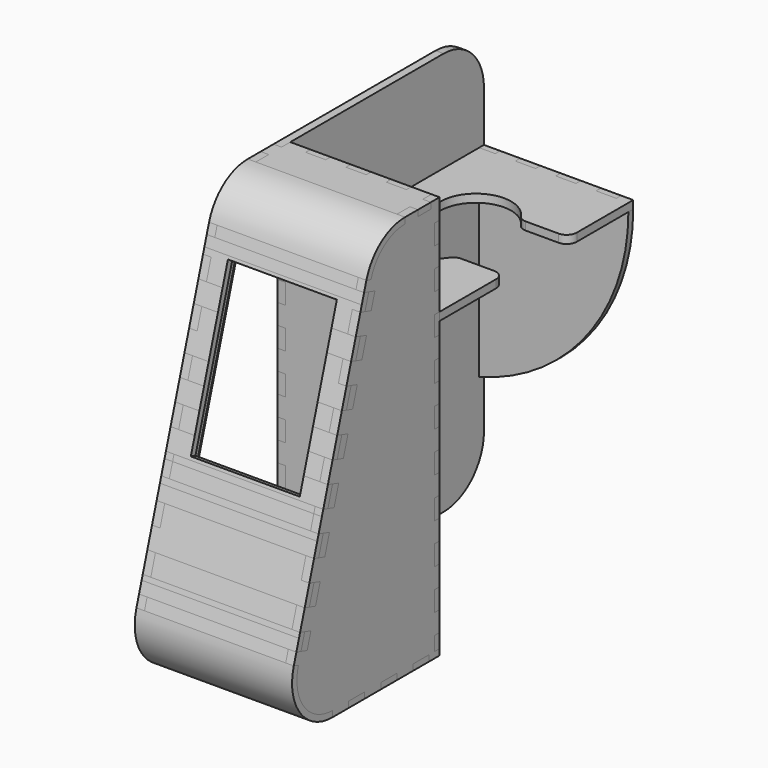
from build123d import *

# Parameters (mm, degrees)
F0_W      = 3
F0_H      = 7
F0_H_2    = 10
F0_R      = 2
F0_W_2    = 10
F0_H_3    = 4
F0_H_4    = 3
F0_W_3    = 2.3992337277
F0_W_4    = 3.3992337277
F1_DEPTH  = 4
F2_DEPTH  = 78
F3_DEPTH  = 78
F0_W_5    = 8
F4_DEPTH  = 78
F5_DEPTH  = 78
F6_START  = 74
F6_DEPTH  = 4
F7_W      = 57
F7_H      = 86.0071991074
F7_W_2    = 54
F7_H_2    = 80.0071991074
F7_W_3    = 59.9
F7_H_3    = 39.3927373791
F8_DEPTH  = 4
F9_DEPTH  = 3
F15_W     = 10
F15_H     = 3
F15_H_2   = 4
F16_DEPTH = 3
F19_W     = 4
F19_H     = 15
F19_H_2   = 10
F19_H_3   = 11
F20_DEPTH = 3
F21_DEPTH = 4
F24_R     = 4
F25_DEPTH = 3
F27_DEPTH = 4


# Not quite as in the source:
# - a feature names something its author has since deleted; it is built from what else it names


with BuildPart() as f1:
    # F0 (on Right) → F1 (new body)
    with BuildSketch(Plane.YZ):
        Polygon((-63.4476184856, 111.4009652057), (-66.3210973413, 112.2630088624), (-69.194576197, 102.6847460101), (-66.3210973413, 101.8227023534), align=None)
        Polygon((-66.3210973413, 101.8227023534), (-62.4897922004, 100.6733108112), (-59.6163133447, 110.2515736634), (-63.4476184856, 111.4009652057), align=None)
        Polygon((-53.8693556334, 129.4080993678), (-57.7006607743, 130.5574909101), (-60.57413963, 120.9792280579), (-56.7428344891, 119.8298365156), align=None)
        Polygon((-51.953703063, 149.7140166145), (-54.8271819186, 150.5760602712), (-57.7006607743, 140.997797419), (-54.8271819186, 140.1357537623), align=None)
        Polygon((-48.1223979221, 148.5646250722), (-51.953703063, 149.7140166145), (-54.8271819186, 140.1357537623), (-50.9958767778, 138.98636222), align=None)
        Polygon((-46.2067453516, 168.8705423189), (-49.0802242073, 169.7325859756), (-51.953703063, 160.1543231234), (-49.0802242073, 159.2922794667), align=None)
        Polygon((-42.3754402108, 167.7211507767), (-46.2067453516, 168.8705423189), (-49.0802242073, 159.2922794667), (-45.2489190664, 158.1428879244), align=None)
        Polygon((-13.3992337277, 197), (-13.3992337277, 200), (-21.3992337277, 200), (-21.3992337277, 198.5), (-21.3992337277, 197), align=None)
        with Locations((-1.5, 193.5)):
            Rectangle(F0_W, F0_H)
        with Locations((-1.5, 175)):
            Rectangle(F0_W, F0_H_2)
        with Locations((-1.5, 155)):
            Rectangle(F0_W, F0_H_2)
        with Locations((-1.5, 135)):
            Rectangle(F0_W, F0_H_2)
        with Locations((-1.5, 115)):
            Rectangle(F0_W, F0_H_2)
        with Locations((-1.5, 95)):
            Rectangle(F0_W, F0_H_2)
        with Locations((-1.5, 75)):
            Rectangle(F0_W, F0_H_2)
        with Locations((-1.5, 55)):
            Rectangle(F0_W, F0_H_2)
        with Locations((-1.5, 35)):
            Rectangle(F0_W, F0_H_2)
        with Locations((-1.5, 15)):
            Rectangle(F0_W, F0_H_2)
        with BuildLine():
            Line((0, 3), (0, 0))
            Line((0, 0), (95, 0))
            ThreePointArc((95, 0), (112.6776695297, 7.3223304703), (120, 25))
            Line((120, 25), (120, 175))
            ThreePointArc((120, 175), (112.6776695297, 192.6776695297), (95, 200))
            Line((95, 200), (0, 200))
            Line((0, 200), (0, 197))
            Line((0, 197), (0, 190))
            Line((0, 190), (0, 180))
            Line((0, 180), (0, 170))
            Line((0, 170), (0, 160))
            Line((0, 160), (0, 150))
            Line((0, 150), (0, 140))
            Line((0, 140), (0, 130))
            Line((0, 130), (0, 120))
            Line((0, 120), (0, 110))
            Line((0, 110), (0, 100))
            Line((0, 100), (0, 90))
            Line((0, 90), (0, 80))
            Line((0, 80), (0, 70))
            Line((0, 70), (0, 60))
            Line((0, 60), (0, 50))
            Line((0, 50), (0, 40))
            Line((0, 40), (0, 30))
            Line((0, 30), (0, 20))
            Line((0, 20), (0, 10))
            Line((0, 10), (0, 3))
        make_face()
        with Locations((95, 25)):
            Circle(F0_R, mode=Mode.SUBTRACT)
        with Locations((10, 148)):
            Rectangle(F0_W_2, F0_H_3, mode=Mode.SUBTRACT)
        with Locations((30, 148)):
            Rectangle(F0_W_2, F0_H_3, mode=Mode.SUBTRACT)
        with Locations((50, 148)):
            Rectangle(F0_W_2, F0_H_3, mode=Mode.SUBTRACT)
        with Locations((70, 148)):
            Rectangle(F0_W_2, F0_H_3, mode=Mode.SUBTRACT)
        with Locations((90, 148)):
            Rectangle(F0_W_2, F0_H_3, mode=Mode.SUBTRACT)
        with Locations((110, 148)):
            Rectangle(F0_W_2, F0_H_3, mode=Mode.SUBTRACT)
        with Locations((95, 175)):
            Circle(F0_R, mode=Mode.SUBTRACT)
        with BuildLine():
            Line((-6.3992337277, 3), (-3, 3))
            Line((-3, 3), (-3, 10))
            Line((-3, 10), (-3, 20))
            Line((-3, 20), (-3, 30))
            Line((-3, 30), (-3, 40))
            Line((-3, 40), (-3, 50))
            Line((-3, 50), (-3, 60))
            Line((-3, 60), (-3, 70))
            Line((-3, 70), (-3, 80))
            Line((-3, 80), (-3, 90))
            Line((-3, 90), (-3, 100))
            Line((-3, 100), (-3, 110))
            Line((-3, 110), (-3, 120))
            Line((-3, 120), (-3, 130))
            Line((-3, 130), (-3, 140))
            Line((-3, 140), (-3, 150))
            Line((-3, 150), (-3, 160))
            Line((-3, 160), (-3, 170))
            Line((-3, 170), (-3, 180))
            Line((-3, 180), (-3, 190))
            Line((-3, 190), (-3, 197))
            Line((-3, 197), (-5.3992337277, 197))
            Line((-5.3992337277, 197), (-13.3992337277, 197))
            Line((-13.3992337277, 197), (-21.3992337277, 197))
            ThreePointArc((-21.3992337277, 197), (-34.5317053798, 192.6504444224), (-42.4714120026, 181.3216534825))
            Line((-42.4714120026, 181.3216534825), (-38.6401068617, 180.1722619402))
            Line((-38.6401068617, 180.1722619402), (-40.0744328665, 175.3911752574))
            Line((-40.0744328665, 175.3911752574), (-42.3754402108, 167.7211507767))
            Line((-42.3754402108, 167.7211507767), (-45.2489190664, 158.1428879244))
            Line((-45.2489190664, 158.1428879244), (-48.1223979221, 148.5646250722))
            Line((-48.1223979221, 148.5646250722), (-50.9958767778, 138.98636222))
            Line((-50.9958767778, 138.98636222), (-53.8693556334, 129.4080993678))
            Line((-53.8693556334, 129.4080993678), (-56.7428344891, 119.8298365156))
            Line((-56.7428344891, 119.8298365156), (-59.6163133447, 110.2515736634))
            Line((-59.6163133447, 110.2515736634), (-62.4897922004, 100.6733108112))
            Line((-62.4897922004, 100.6733108112), (-65.3632710561, 91.095047959))
            Line((-65.3632710561, 91.095047959), (-68.2367499117, 81.5167851068))
            Line((-68.2367499117, 81.5167851068), (-71.1102287674, 71.9385222545))
            Line((-71.1102287674, 71.9385222545), (-73.9837076231, 62.3602594023))
            Line((-73.9837076231, 62.3602594023), (-76.8571864787, 52.7819965501))
            Line((-76.8571864787, 52.7819965501), (-79.7306653344, 43.2037336979))
            Line((-79.7306653344, 43.2037336979), (-82.0278634272, 35.546406722))
            Line((-82.0278634272, 35.546406722), (-83.6401068617, 30.1722619402))
            Line((-83.6401068617, 30.1722619402), (-87.4714120026, 31.3216534825))
            ThreePointArc((-87.4714120026, 31.3216534825), (-84.0496781501, 11.8675283479), (-66.3992337277, 3))
            Line((-66.3992337277, 3), (-56.3992337277, 3))
            Line((-56.3992337277, 3), (-46.3992337277, 3))
            Line((-46.3992337277, 3), (-36.3992337277, 3))
            Line((-36.3992337277, 3), (-26.3992337277, 3))
            Line((-26.3992337277, 3), (-16.3992337277, 3))
            Line((-16.3992337277, 3), (-6.3992337277, 3))
        make_face()
        with Locations((-66.3992337277, 25)):
            Circle(F0_R, mode=Mode.SUBTRACT)
        with Locations((-21.3992337277, 175)):
            Circle(F0_R, mode=Mode.SUBTRACT)
        Polygon((-38.6401068617, 180.1722619402), (-42.4714120026, 181.3216534825), (-43.9071171063, 176.5359698035), (-40.0744328665, 175.3911752574), align=None)
        with Locations((-1.5, 1.5)):
            Rectangle(F0_W, F0_H_4)
        with Locations((-1.5, 198.5)):
            Rectangle(F0_W, F0_H_4)
        with Locations((-4.1996168639, 198.5)):
            Rectangle(F0_W_3, F0_H_4)
        Polygon((-72.0680550526, 82.666176649), (-68.2367499117, 81.5167851068), (-65.3632710561, 91.095047959), (-69.194576197, 92.2444395012), (-70.056809017, 89.3703301012), align=None)
        Polygon((-77.8150127639, 73.9499574535), (-80.6884916196, 64.3716946013), (-77.8150127639, 63.5096509446), (-74.9415339083, 73.0879137968), align=None)
        Polygon((-74.9415339083, 73.0879137968), (-77.8150127639, 63.5096509446), (-73.9837076231, 62.3602594023), (-71.1102287674, 71.9385222545), align=None)
        Polygon((-83.5619704753, 54.7934317491), (-86.4354493309, 45.2151688969), (-83.5619704753, 44.3531252402), (-80.6884916196, 53.9313880924), align=None)
        Polygon((-80.6884916196, 53.9313880924), (-83.5619704753, 44.3531252402), (-79.7306653344, 43.2037336979), (-76.8571864787, 52.7819965501), align=None)
        Polygon((-88.7350821389, 37.5497262036), (-90.3448908583, 32.1836971392), (-87.4714120026, 31.3216534825), (-85.8605598339, 36.6911607115), align=None)
        Polygon((-85.8605598339, 36.6911607115), (-87.4714120026, 31.3216534825), (-83.6401068617, 30.1722619402), (-82.0278634272, 35.546406722), align=None)
        Polygon((-43.9081514304, 181.7526753108), (-45.3448908583, 182.1836971392), (-46.7816302861, 177.3945657131), (-43.9071171063, 176.5359698035), (-42.4714120026, 181.3216534825), align=None)
        Polygon((-57.7006607743, 130.5574909101), (-60.57413963, 131.4195345668), (-63.4476184856, 121.8412717146), (-60.57413963, 120.9792280579), align=None)
        Polygon((-72.9302878726, 90.2323737579), (-74.9415339083, 83.5282203057), (-72.0680550526, 82.666176649), (-70.056809017, 89.3703301012), (-69.194576197, 92.2444395012), (-72.0680550526, 93.1064831579), align=None)
        with Locations((-4.6996168639, 1.5)):
            Rectangle(F0_W_4, F0_H_4)
        with Locations((-21.3992337277, 1.5)):
            Rectangle(F0_W_2, F0_H_4)
        with Locations((-41.3992337277, 1.5)):
            Rectangle(F0_W_2, F0_H_4)
        with Locations((-61.3992337277, 1.5)):
            Rectangle(F0_W_2, F0_H_4)
        with Locations((-21.3992337277, 175)):
            Circle(F0_R)
        with Locations((-66.3992337277, 25)):
            Circle(F0_R)
        with Locations((95, 25)):
            Circle(F0_R)
        with Locations((95, 175)):
            Circle(F0_R)
    extrude(amount=F1_DEPTH)


with BuildPart() as f2:
    # F0 (on Right) → F2 (new body)
    with BuildSketch(Plane.YZ):
        with Locations((-1.5, 193.5)):
            Rectangle(F0_W, F0_H)
        with Locations((-1.5, 185)):
            Rectangle(F0_W, F0_H_2)
        with Locations((-1.5, 175)):
            Rectangle(F0_W, F0_H_2)
        with Locations((-1.5, 165)):
            Rectangle(F0_W, F0_H_2)
        with Locations((-1.5, 155)):
            Rectangle(F0_W, F0_H_2)
        with Locations((-1.5, 145)):
            Rectangle(F0_W, F0_H_2)
        with Locations((-1.5, 135)):
            Rectangle(F0_W, F0_H_2)
        with Locations((-1.5, 125)):
            Rectangle(F0_W, F0_H_2)
        with Locations((-1.5, 115)):
            Rectangle(F0_W, F0_H_2)
        with Locations((-1.5, 105)):
            Rectangle(F0_W, F0_H_2)
        with Locations((-1.5, 95)):
            Rectangle(F0_W, F0_H_2)
        with Locations((-1.5, 85)):
            Rectangle(F0_W, F0_H_2)
        with Locations((-1.5, 75)):
            Rectangle(F0_W, F0_H_2)
        with Locations((-1.5, 65)):
            Rectangle(F0_W, F0_H_2)
        with Locations((-1.5, 55)):
            Rectangle(F0_W, F0_H_2)
        with Locations((-1.5, 45)):
            Rectangle(F0_W, F0_H_2)
        with Locations((-1.5, 35)):
            Rectangle(F0_W, F0_H_2)
        with Locations((-1.5, 25)):
            Rectangle(F0_W, F0_H_2)
        with Locations((-1.5, 15)):
            Rectangle(F0_W, F0_H_2)
        with Locations((-1.5, 6.5)):
            Rectangle(F0_W, F0_H)
        with Locations((-1.5, 198.5)):
            Rectangle(F0_W, F0_H_4)
        with Locations((-1.5, 1.5)):
            Rectangle(F0_W, F0_H_4)
    extrude(amount=F2_DEPTH)


with BuildPart() as f3:
    # F0 (on Right) → F3 (new body)
    with BuildSketch(Plane.YZ):
        Polygon((-88.7350821389, 37.5497262036), (-90.3448908583, 32.1836971392), (-87.4714120026, 31.3216534825), (-85.8605598339, 36.6911607115), align=None)
        with Locations((-1.5, 1.5)):
            Rectangle(F0_W, F0_H_4)
        with BuildLine():
            ThreePointArc((-90.3448908583, 32.1836971392), (-86.456556935, 10.076736759), (-66.3992337277, 0))
            Line((-66.3992337277, 0), (-66.3992337277, 3))
            ThreePointArc((-66.3992337277, 3), (-84.0496781501, 11.8675283479), (-87.4714120026, 31.3216534825))
            Line((-87.4714120026, 31.3216534825), (-90.3448908583, 32.1836971392))
        make_face()
        with Locations((-4.6996168639, 1.5)):
            Rectangle(F0_W_4, F0_H_4)
        with Locations((-11.3992337277, 1.5)):
            Rectangle(F0_W_2, F0_H_4)
        with Locations((-21.3992337277, 1.5)):
            Rectangle(F0_W_2, F0_H_4)
        with Locations((-31.3992337277, 1.5)):
            Rectangle(F0_W_2, F0_H_4)
        with Locations((-41.3992337277, 1.5)):
            Rectangle(F0_W_2, F0_H_4)
        with Locations((-51.3992337277, 1.5)):
            Rectangle(F0_W_2, F0_H_4)
        with Locations((-61.3992337277, 1.5)):
            Rectangle(F0_W_2, F0_H_4)
    extrude(amount=F3_DEPTH)


with BuildPart() as f3b:
    # F0 (on Right) → F3, piece 2 (new body)
    with BuildSketch(Plane.YZ):
        Polygon((-13.3992337277, 197), (-13.3992337277, 200), (-21.3992337277, 200), (-21.3992337277, 198.5), (-21.3992337277, 197), align=None)
        with Locations((-9.3992337277, 198.5)):
            Rectangle(F0_W_5, F0_H_4)
        with Locations((-4.1996168639, 198.5)):
            Rectangle(F0_W_3, F0_H_4)
        with Locations((-1.5, 198.5)):
            Rectangle(F0_W, F0_H_4)
        with BuildLine():
            Line((-21.3992337277, 198.5), (-21.3992337277, 200))
            ThreePointArc((-21.3992337277, 200), (-36.3224969687, 195.0573232072), (-45.3448908583, 182.1836971392))
            Line((-45.3448908583, 182.1836971392), (-43.9081514304, 181.7526753108))
            Line((-43.9081514304, 181.7526753108), (-42.4714120026, 181.3216534825))
            ThreePointArc((-42.4714120026, 181.3216534825), (-34.5317053798, 192.6504444224), (-21.3992337277, 197))
            Line((-21.3992337277, 197), (-21.3992337277, 198.5))
        make_face()
        Polygon((-43.9081514304, 181.7526753108), (-45.3448908583, 182.1836971392), (-46.7816302861, 177.3945657131), (-43.9071171063, 176.5359698035), (-42.4714120026, 181.3216534825), align=None)
    extrude(amount=F3_DEPTH)


with BuildPart() as f4:
    # F0 (on Right) → F4 (new body)
    with BuildSketch(Plane.YZ):
        Polygon((-77.8150127639, 73.9499574535), (-80.6884916196, 64.3716946013), (-77.8150127639, 63.5096509446), (-74.9415339083, 73.0879137968), align=None)
        Polygon((-69.194576197, 102.6847460101), (-72.0680550526, 93.1064831579), (-69.194576197, 92.2444395012), (-66.3210973413, 101.8227023534), align=None)
        Polygon((-63.4476184856, 111.4009652057), (-66.3210973413, 112.2630088624), (-69.194576197, 102.6847460101), (-66.3210973413, 101.8227023534), align=None)
        Polygon((-60.57413963, 120.9792280579), (-63.4476184856, 121.8412717146), (-66.3210973413, 112.2630088624), (-63.4476184856, 111.4009652057), align=None)
        Polygon((-57.7006607743, 130.5574909101), (-60.57413963, 131.4195345668), (-63.4476184856, 121.8412717146), (-60.57413963, 120.9792280579), align=None)
        Polygon((-54.8271819186, 140.1357537623), (-57.7006607743, 140.997797419), (-60.57413963, 131.4195345668), (-57.7006607743, 130.5574909101), align=None)
        Polygon((-51.953703063, 149.7140166145), (-54.8271819186, 150.5760602712), (-57.7006607743, 140.997797419), (-54.8271819186, 140.1357537623), align=None)
        Polygon((-49.0802242073, 159.2922794667), (-51.953703063, 160.1543231234), (-54.8271819186, 150.5760602712), (-51.953703063, 149.7140166145), align=None)
        Polygon((-46.2067453516, 168.8705423189), (-49.0802242073, 169.7325859756), (-51.953703063, 160.1543231234), (-49.0802242073, 159.2922794667), align=None)
        Polygon((-45.34282221, 171.7502861245), (-48.2183697139, 172.6054342869), (-49.0802242073, 169.7325859756), (-46.2067453516, 168.8705423189), align=None)
        Polygon((-80.6884916196, 64.3716946013), (-83.5619704753, 54.7934317491), (-80.6884916196, 53.9313880924), (-77.8150127639, 63.5096509446), align=None)
        Polygon((-83.5619704753, 54.7934317491), (-86.4354493309, 45.2151688969), (-83.5619704753, 44.3531252402), (-80.6884916196, 53.9313880924), align=None)
        Polygon((-86.4354493309, 45.2151688969), (-87.1252734196, 42.915755268), (-84.2497076652, 42.0606679405), (-83.5619704753, 44.3531252402), align=None)
        Polygon((-87.1252734196, 42.915755268), (-88.7350821389, 37.5497262036), (-85.8605598339, 36.6911607115), (-84.2497076652, 42.0606679405), align=None)
        Polygon((-43.9071171063, 176.5359698035), (-46.7816302861, 177.3945657131), (-48.2183697139, 172.6054342869), (-45.34282221, 171.7502861245), align=None)
        Polygon((-75.8037667283, 80.6541109057), (-77.8150127639, 73.9499574535), (-74.9415339083, 73.0879137968), (-72.9302878726, 79.792067249), (-72.0680550526, 82.666176649), (-74.9415339083, 83.5282203057), align=None)
        Polygon((-72.9302878726, 90.2323737579), (-74.9415339083, 83.5282203057), (-72.0680550526, 82.666176649), (-70.056809017, 89.3703301012), (-69.194576197, 92.2444395012), (-72.0680550526, 93.1064831579), align=None)
    extrude(amount=F4_DEPTH)

    # F7 (on face) → F9 (cut)
    with BuildSketch(Plane(origin=(0, -88.8696404104, 26.6608921231), x_dir=(1, 0, 0), z_dir=(0, -0.9578262852, 0.2873478856))):
        with Locations((39, 109.974174903)):
            Rectangle(F7_W_2, F7_H_2)
    extrude(amount=F9_DEPTH, mode=Mode.SUBTRACT)


with BuildPart() as f5:
    # F0 (on Right) → F5 (new body)
    with BuildSketch(Plane.YZ):
        Polygon((-38.6401068617, 180.1722619402), (-42.4714120026, 181.3216534825), (-43.9071171063, 176.5359698035), (-40.0744328665, 175.3911752574), align=None)
        Polygon((-40.0744328665, 175.3911752574), (-43.9071171063, 176.5359698035), (-45.34282221, 171.7502861245), (-46.2067453516, 168.8705423189), (-42.3754402108, 167.7211507767), align=None)
        Polygon((-42.3754402108, 167.7211507767), (-46.2067453516, 168.8705423189), (-49.0802242073, 159.2922794667), (-45.2489190664, 158.1428879244), align=None)
        Polygon((-45.2489190664, 158.1428879244), (-49.0802242073, 159.2922794667), (-51.953703063, 149.7140166145), (-48.1223979221, 148.5646250722), align=None)
        Polygon((-48.1223979221, 148.5646250722), (-51.953703063, 149.7140166145), (-54.8271819186, 140.1357537623), (-50.9958767778, 138.98636222), align=None)
        Polygon((-50.9958767778, 138.98636222), (-54.8271819186, 140.1357537623), (-57.7006607743, 130.5574909101), (-53.8693556334, 129.4080993678), align=None)
        Polygon((-53.8693556334, 129.4080993678), (-57.7006607743, 130.5574909101), (-60.57413963, 120.9792280579), (-56.7428344891, 119.8298365156), align=None)
        Polygon((-56.7428344891, 119.8298365156), (-60.57413963, 120.9792280579), (-63.4476184856, 111.4009652057), (-59.6163133447, 110.2515736634), align=None)
        Polygon((-66.3210973413, 101.8227023534), (-62.4897922004, 100.6733108112), (-59.6163133447, 110.2515736634), (-63.4476184856, 111.4009652057), align=None)
        Polygon((-69.194576197, 92.2444395012), (-65.3632710561, 91.095047959), (-62.4897922004, 100.6733108112), (-66.3210973413, 101.8227023534), align=None)
        Polygon((-72.0680550526, 82.666176649), (-68.2367499117, 81.5167851068), (-65.3632710561, 91.095047959), (-69.194576197, 92.2444395012), (-70.056809017, 89.3703301012), align=None)
        Polygon((-72.9302878726, 79.792067249), (-74.9415339083, 73.0879137968), (-71.1102287674, 71.9385222545), (-68.2367499117, 81.5167851068), (-72.0680550526, 82.666176649), align=None)
        Polygon((-74.9415339083, 73.0879137968), (-77.8150127639, 63.5096509446), (-73.9837076231, 62.3602594023), (-71.1102287674, 71.9385222545), align=None)
        Polygon((-77.8150127639, 63.5096509446), (-80.6884916196, 53.9313880924), (-76.8571864787, 52.7819965501), (-73.9837076231, 62.3602594023), align=None)
        Polygon((-80.6884916196, 53.9313880924), (-83.5619704753, 44.3531252402), (-79.7306653344, 43.2037336979), (-76.8571864787, 52.7819965501), align=None)
        Polygon((-84.2497076652, 42.0606679405), (-85.8605598339, 36.6911607115), (-82.0278634272, 35.546406722), (-79.7306653344, 43.2037336979), (-83.5619704753, 44.3531252402), align=None)
        Polygon((-85.8605598339, 36.6911607115), (-87.4714120026, 31.3216534825), (-83.6401068617, 30.1722619402), (-82.0278634272, 35.546406722), align=None)
    extrude(amount=F5_DEPTH)

    # F7 (on face) → F8 (cut)
    with BuildSketch(Plane(origin=(0, -88.8696404104, 26.6608921231), x_dir=(1, 0, 0), z_dir=(0, -0.9578262852, 0.2873478856))):
        with Locations((39, 108.474174903)):
            Rectangle(F7_W, F7_H)
        with Locations((39, 109.974174903)):
            Rectangle(F7_W_2, F7_H_2, mode=Mode.SUBTRACT)
        with Locations((39, 109.974174903)):
            Rectangle(F7_W_2, F7_H_2)
        with Locations((39, 35.7742066597)):
            Rectangle(F7_W_3, F7_H_3)
    extrude(amount=-F8_DEPTH, mode=Mode.SUBTRACT)


with BuildPart() as f6:
    # F0 (on Right) → F6 (new body)
    with BuildSketch(Plane.YZ.offset(F6_START)):
        Polygon((-63.4476184856, 111.4009652057), (-66.3210973413, 112.2630088624), (-69.194576197, 102.6847460101), (-66.3210973413, 101.8227023534), align=None)
        Polygon((-66.3210973413, 101.8227023534), (-62.4897922004, 100.6733108112), (-59.6163133447, 110.2515736634), (-63.4476184856, 111.4009652057), align=None)
        Polygon((-53.8693556334, 129.4080993678), (-57.7006607743, 130.5574909101), (-60.57413963, 120.9792280579), (-56.7428344891, 119.8298365156), align=None)
        Polygon((-51.953703063, 149.7140166145), (-54.8271819186, 150.5760602712), (-57.7006607743, 140.997797419), (-54.8271819186, 140.1357537623), align=None)
        Polygon((-48.1223979221, 148.5646250722), (-51.953703063, 149.7140166145), (-54.8271819186, 140.1357537623), (-50.9958767778, 138.98636222), align=None)
        Polygon((-46.2067453516, 168.8705423189), (-49.0802242073, 169.7325859756), (-51.953703063, 160.1543231234), (-49.0802242073, 159.2922794667), align=None)
        Polygon((-42.3754402108, 167.7211507767), (-46.2067453516, 168.8705423189), (-49.0802242073, 159.2922794667), (-45.2489190664, 158.1428879244), align=None)
        Polygon((-13.3992337277, 197), (-13.3992337277, 200), (-21.3992337277, 200), (-21.3992337277, 198.5), (-21.3992337277, 197), align=None)
        with Locations((-1.5, 193.5)):
            Rectangle(F0_W, F0_H)
        with Locations((-1.5, 175)):
            Rectangle(F0_W, F0_H_2)
        with Locations((-1.5, 155)):
            Rectangle(F0_W, F0_H_2)
        with Locations((-1.5, 135)):
            Rectangle(F0_W, F0_H_2)
        with Locations((-1.5, 115)):
            Rectangle(F0_W, F0_H_2)
        with Locations((-1.5, 95)):
            Rectangle(F0_W, F0_H_2)
        with Locations((-1.5, 75)):
            Rectangle(F0_W, F0_H_2)
        with Locations((-1.5, 55)):
            Rectangle(F0_W, F0_H_2)
        with Locations((-1.5, 35)):
            Rectangle(F0_W, F0_H_2)
        with Locations((-1.5, 15)):
            Rectangle(F0_W, F0_H_2)
        with BuildLine():
            Line((-6.3992337277, 3), (-3, 3))
            Line((-3, 3), (-3, 10))
            Line((-3, 10), (-3, 20))
            Line((-3, 20), (-3, 30))
            Line((-3, 30), (-3, 40))
            Line((-3, 40), (-3, 50))
            Line((-3, 50), (-3, 60))
            Line((-3, 60), (-3, 70))
            Line((-3, 70), (-3, 80))
            Line((-3, 80), (-3, 90))
            Line((-3, 90), (-3, 100))
            Line((-3, 100), (-3, 110))
            Line((-3, 110), (-3, 120))
            Line((-3, 120), (-3, 130))
            Line((-3, 130), (-3, 140))
            Line((-3, 140), (-3, 150))
            Line((-3, 150), (-3, 160))
            Line((-3, 160), (-3, 170))
            Line((-3, 170), (-3, 180))
            Line((-3, 180), (-3, 190))
            Line((-3, 190), (-3, 197))
            Line((-3, 197), (-5.3992337277, 197))
            Line((-5.3992337277, 197), (-13.3992337277, 197))
            Line((-13.3992337277, 197), (-21.3992337277, 197))
            ThreePointArc((-21.3992337277, 197), (-34.5317053798, 192.6504444224), (-42.4714120026, 181.3216534825))
            Line((-42.4714120026, 181.3216534825), (-38.6401068617, 180.1722619402))
            Line((-38.6401068617, 180.1722619402), (-40.0744328665, 175.3911752574))
            Line((-40.0744328665, 175.3911752574), (-42.3754402108, 167.7211507767))
            Line((-42.3754402108, 167.7211507767), (-45.2489190664, 158.1428879244))
            Line((-45.2489190664, 158.1428879244), (-48.1223979221, 148.5646250722))
            Line((-48.1223979221, 148.5646250722), (-50.9958767778, 138.98636222))
            Line((-50.9958767778, 138.98636222), (-53.8693556334, 129.4080993678))
            Line((-53.8693556334, 129.4080993678), (-56.7428344891, 119.8298365156))
            Line((-56.7428344891, 119.8298365156), (-59.6163133447, 110.2515736634))
            Line((-59.6163133447, 110.2515736634), (-62.4897922004, 100.6733108112))
            Line((-62.4897922004, 100.6733108112), (-65.3632710561, 91.095047959))
            Line((-65.3632710561, 91.095047959), (-68.2367499117, 81.5167851068))
            Line((-68.2367499117, 81.5167851068), (-71.1102287674, 71.9385222545))
            Line((-71.1102287674, 71.9385222545), (-73.9837076231, 62.3602594023))
            Line((-73.9837076231, 62.3602594023), (-76.8571864787, 52.7819965501))
            Line((-76.8571864787, 52.7819965501), (-79.7306653344, 43.2037336979))
            Line((-79.7306653344, 43.2037336979), (-82.0278634272, 35.546406722))
            Line((-82.0278634272, 35.546406722), (-83.6401068617, 30.1722619402))
            Line((-83.6401068617, 30.1722619402), (-87.4714120026, 31.3216534825))
            ThreePointArc((-87.4714120026, 31.3216534825), (-84.0496781501, 11.8675283479), (-66.3992337277, 3))
            Line((-66.3992337277, 3), (-56.3992337277, 3))
            Line((-56.3992337277, 3), (-46.3992337277, 3))
            Line((-46.3992337277, 3), (-36.3992337277, 3))
            Line((-36.3992337277, 3), (-26.3992337277, 3))
            Line((-26.3992337277, 3), (-16.3992337277, 3))
            Line((-16.3992337277, 3), (-6.3992337277, 3))
        make_face()
        with Locations((-66.3992337277, 25)):
            Circle(F0_R, mode=Mode.SUBTRACT)
        with Locations((-21.3992337277, 175)):
            Circle(F0_R, mode=Mode.SUBTRACT)
        Polygon((-38.6401068617, 180.1722619402), (-42.4714120026, 181.3216534825), (-43.9071171063, 176.5359698035), (-40.0744328665, 175.3911752574), align=None)
        with Locations((-1.5, 1.5)):
            Rectangle(F0_W, F0_H_4)
        with Locations((-21.3992337277, 175)):
            Circle(F0_R)
        with Locations((-66.3992337277, 25)):
            Circle(F0_R)
        with Locations((-1.5, 198.5)):
            Rectangle(F0_W, F0_H_4)
        with Locations((-4.1996168639, 198.5)):
            Rectangle(F0_W_3, F0_H_4)
        Polygon((-72.9302878726, 90.2323737579), (-74.9415339083, 83.5282203057), (-72.0680550526, 82.666176649), (-70.056809017, 89.3703301012), (-69.194576197, 92.2444395012), (-72.0680550526, 93.1064831579), align=None)
        Polygon((-72.0680550526, 82.666176649), (-68.2367499117, 81.5167851068), (-65.3632710561, 91.095047959), (-69.194576197, 92.2444395012), (-70.056809017, 89.3703301012), align=None)
        Polygon((-77.8150127639, 73.9499574535), (-80.6884916196, 64.3716946013), (-77.8150127639, 63.5096509446), (-74.9415339083, 73.0879137968), align=None)
        Polygon((-74.9415339083, 73.0879137968), (-77.8150127639, 63.5096509446), (-73.9837076231, 62.3602594023), (-71.1102287674, 71.9385222545), align=None)
        Polygon((-83.5619704753, 54.7934317491), (-86.4354493309, 45.2151688969), (-83.5619704753, 44.3531252402), (-80.6884916196, 53.9313880924), align=None)
        Polygon((-80.6884916196, 53.9313880924), (-83.5619704753, 44.3531252402), (-79.7306653344, 43.2037336979), (-76.8571864787, 52.7819965501), align=None)
        Polygon((-88.7350821389, 37.5497262036), (-90.3448908583, 32.1836971392), (-87.4714120026, 31.3216534825), (-85.8605598339, 36.6911607115), align=None)
        Polygon((-85.8605598339, 36.6911607115), (-87.4714120026, 31.3216534825), (-83.6401068617, 30.1722619402), (-82.0278634272, 35.546406722), align=None)
        Polygon((-43.9081514304, 181.7526753108), (-45.3448908583, 182.1836971392), (-46.7816302861, 177.3945657131), (-43.9071171063, 176.5359698035), (-42.4714120026, 181.3216534825), align=None)
        Polygon((-57.7006607743, 130.5574909101), (-60.57413963, 131.4195345668), (-63.4476184856, 121.8412717146), (-60.57413963, 120.9792280579), align=None)
        with Locations((-41.3992337277, 1.5)):
            Rectangle(F0_W_2, F0_H_4)
        with Locations((-61.3992337277, 1.5)):
            Rectangle(F0_W_2, F0_H_4)
        with Locations((-21.3992337277, 1.5)):
            Rectangle(F0_W_2, F0_H_4)
        with Locations((-4.6996168639, 1.5)):
            Rectangle(F0_W_4, F0_H_4)
    extrude(amount=F6_DEPTH)


with BuildPart() as f2_1:
    add(f2.part)

    # F10: cut F1, F6
    add(f1.part, mode=Mode.SUBTRACT)
    add(f6.part, mode=Mode.SUBTRACT)

    # F15 (on face) → F16 (cut)
    with BuildSketch(Plane(origin=(0, 0, 0), x_dir=(-1, 0, 0), z_dir=(0, 1, 0))):
        with Locations((-69, 198.5)):
            Rectangle(F15_W, F15_H)
        with Locations((-69, 1.5)):
            Rectangle(F15_W, F15_H)
        with Locations((-49, 198.5)):
            Rectangle(F15_W, F15_H)
        with Locations((-49, 1.5)):
            Rectangle(F15_W, F15_H)
        with Locations((-29, 198.5)):
            Rectangle(F15_W, F15_H)
        with Locations((-29, 1.5)):
            Rectangle(F15_W, F15_H)
        with Locations((-9, 198.5)):
            Rectangle(F15_W, F15_H)
        with Locations((-9, 1.5)):
            Rectangle(F15_W, F15_H)
        with Locations((-59, 148)):
            Rectangle(F15_W, F15_H_2)
        with Locations((-39, 148)):
            Rectangle(F15_W, F15_H_2)
        with Locations((-19, 148)):
            Rectangle(F15_W, F15_H_2)
    extrude(amount=-F16_DEPTH, mode=Mode.SUBTRACT)


with BuildPart() as f3b_1:
    add(f3b.part)

    # F11: cut F6, F1
    add(f6.part, mode=Mode.SUBTRACT)
    add(f1.part, mode=Mode.SUBTRACT)

    # F17: cut F2
    add(f2_1.part, mode=Mode.SUBTRACT)


with BuildPart() as f4_1:
    add(f4.part)

    # F12: cut F1, F6
    add(f1.part, mode=Mode.SUBTRACT)
    add(f6.part, mode=Mode.SUBTRACT)


with BuildPart() as f5_1:
    add(f5.part)

    # F13: cut F1, F6
    add(f1.part, mode=Mode.SUBTRACT)
    add(f6.part, mode=Mode.SUBTRACT)


with BuildPart() as f3_1:
    add(f3.part)

    # F14: cut F1, F6
    add(f1.part, mode=Mode.SUBTRACT)
    add(f6.part, mode=Mode.SUBTRACT)

    # F17: cut F2
    add(f2_1.part, mode=Mode.SUBTRACT)

    # F24 (on face) → F25 (cut)
    with BuildSketch(Plane(origin=(0, 0, 0), x_dir=(1, 0, 0), z_dir=(0, 0, -1))):
        with BuildLine():
            Line((17, 9), (11, 9))
            ThreePointArc((11, 9), (8, 6), (11, 3))
            Line((11, 3), (14, 3))
            Line((14, 3), (20, 3))
            Line((20, 3), (20, 6))
            ThreePointArc((20, 6), (19.1213203436, 8.1213203436), (17, 9))
        make_face()
        with Locations((11, 16)):
            Circle(F24_R)
    extrude(amount=-F25_DEPTH, mode=Mode.SUBTRACT)


with BuildPart() as f20:
    # F19 (on face) → F20 (new body)
    with BuildSketch(Plane(origin=(0, 120, 0), x_dir=(-1, 0, 0), z_dir=(0, 1, 0))):
        with Locations((-2, 57.5)):
            Rectangle(F19_W, F19_H)
        with Locations((-2, 80)):
            Rectangle(F19_W, F19_H_2)
        with Locations((-2, 100)):
            Rectangle(F19_W, F19_H_2)
        with Locations((-2, 120)):
            Rectangle(F19_W, F19_H_2)
        with Locations((-2, 140.5)):
            Rectangle(F19_W, F19_H_3)
        with BuildLine():
            Line((-4, 146), (-4, 150))
            Line((-4, 150), (-12, 150))
            Line((-12, 150), (-12, 146))
            Line((-12, 146), (-22, 146))
            Line((-22, 146), (-22, 150))
            Line((-22, 150), (-32, 150))
            Line((-32, 150), (-32, 146))
            Line((-32, 146), (-42, 146))
            Line((-42, 146), (-42, 150))
            Line((-42, 150), (-52, 150))
            Line((-52, 150), (-52, 146))
            Line((-52, 146), (-62, 146))
            Line((-62, 146), (-62, 150))
            Line((-62, 150), (-72, 150))
            Line((-72, 150), (-72, 146))
            Line((-72, 146), (-78, 146))
            ThreePointArc((-78, 146), (-57.3527960623, 85.394719702), (-4, 50))
            Line((-4, 50), (-4, 65))
            Line((-4, 65), (-4, 75))
            Line((-4, 75), (-4, 85))
            Line((-4, 85), (-4, 95))
            Line((-4, 95), (-4, 105))
            Line((-4, 105), (-4, 115))
            Line((-4, 115), (-4, 125))
            Line((-4, 125), (-4, 135))
            Line((-4, 135), (-4, 146))
        make_face()
    extrude(amount=-F20_DEPTH)


with BuildPart() as f21:
    # F18 (on face) → F21 (new body)
    with BuildSketch(Plane.XY.offset(146)):
        with BuildLine():
            Line((78, 120), (0, 120))
            Line((0, 120), (0, -3))
            Line((0, -3), (78, -3))
            Line((78, -3), (78, 35))
            ThreePointArc((78, 35), (76.5355339059, 38.5355339059), (73, 40))
            Line((73, 40), (56.7082869339, 40))
            ThreePointArc((56.7082869339, 40), (54.3512643299, 39.4095855184), (52.5508898375, 37.7777777778))
            ThreePointArc((52.5508898375, 37.7777777778), (32.9201659552, 30.7534992886), (20.5, 47.5))
            Line((20.5, 47.5), (20.5, 72.5))
            ThreePointArc((20.5, 72.5), (32.9201659552, 89.2465007114), (52.5508898375, 82.2222222222))
            ThreePointArc((52.5508898375, 82.2222222222), (54.3512643299, 80.5904144816), (56.7082869339, 80))
            Line((56.7082869339, 80), (73, 80))
            ThreePointArc((73, 80), (76.5355339059, 81.4644660941), (78, 85))
            Line((78, 85), (78, 120))
        make_face()
    extrude(amount=F21_DEPTH)


with BuildPart() as f1_1:
    add(f1.part)

    # F22: cut F20
    add(f20.part, mode=Mode.SUBTRACT)


with BuildPart() as f21_1:
    add(f21.part)

    # F23: cut F2, F1, F20
    add(f2_1.part, mode=Mode.SUBTRACT)
    add(f1_1.part, mode=Mode.SUBTRACT)
    add(f20.part, mode=Mode.SUBTRACT)


with BuildPart() as f1_2:
    add(f1_1.part)

    # F26 (on face) → F27 (cut)
    with BuildSketch(Plane.YZ.offset(4)):
        with BuildLine():
            ThreePointArc((-21.3992337277, 183), (-26.1746779648, 181.4183434263), (-29.0618440095, 177.2987830845))
            Line((-29.0618440095, 177.2987830845), (-74.0618440095, 27.2987830845))
            ThreePointArc((-74.0618440095, 27.2987830845), (-72.817577154, 20.2245557629), (-66.3992337277, 17))
            Line((-66.3992337277, 17), (-11, 17))
            ThreePointArc((-11, 17), (-5.3431457505, 19.3431457505), (-3, 25))
            Line((-3, 25), (-3, 30))
            Line((-3, 30), (-3, 40))
            Line((-3, 40), (-3, 50))
            Line((-3, 50), (-3, 60))
            Line((-3, 60), (-3, 70))
            Line((-3, 70), (-3, 80))
            Line((-3, 80), (-3, 90))
            Line((-3, 90), (-3, 100))
            Line((-3, 100), (-3, 110))
            Line((-3, 110), (-3, 120))
            Line((-3, 120), (-3, 130))
            Line((-3, 130), (-3, 140))
            Line((-3, 140), (-3, 150))
            Line((-3, 150), (-3, 160))
            Line((-3, 160), (-3, 170))
            Line((-3, 170), (-3, 175))
            ThreePointArc((-3, 175), (-5.3431457505, 180.6568542495), (-11, 183))
            Line((-11, 183), (-21.3992337277, 183))
        make_face()
    extrude(amount=-F27_DEPTH, mode=Mode.SUBTRACT)


solid = Compound([f6.part, f2_1.part, f3b_1.part, f4_1.part, f5_1.part, f3_1.part, f20.part, f21_1.part, f1_2.part])
